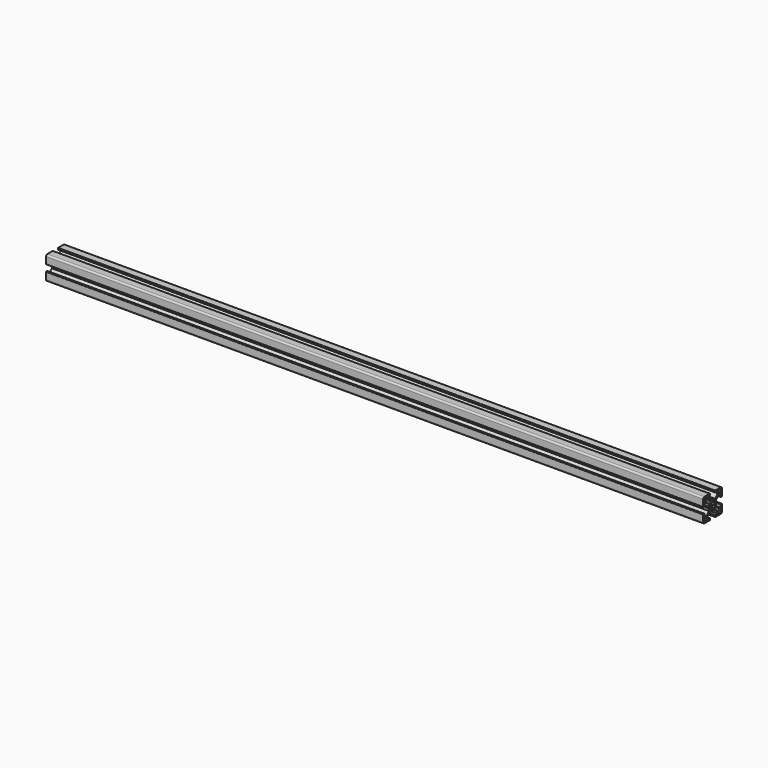
from build123d import *

# Parameters (mm, degrees)
F1_DEPTH = 420


# Not quite as in the source:
# - ends of sketch curves that miss each other by under 0.0002 mm in the source are joined


with BuildPart() as f1:
    # F0 (on Right) → F1 (new body, symmetric)
    with BuildSketch(Plane.YZ):
        with BuildLine():
            Line((14.49994, -4), (13.242475, -4))
            ThreePointArc((13.242475, -4), (12.8889216094, -4.1464466094), (12.742475, -4.5))
            Line((12.742475, -4.5), (12.742475, -7.732519))
            ThreePointArc((12.742475, -7.732519), (12.602449566, -8.0972966877), (12.242781, -8.249967))
            Line((12.242781, -8.249967), (10.260188, -8.249967))
            ThreePointArc((10.260188, -8.249967), (10.0688470492, -8.2119069185), (9.9066360236, -8.1035209764))
            Line((9.9066360236, -8.1035209764), (5.981118, -4.178003))
            ThreePointArc((5.981118, -4.178003), (5.8727320815, -4.0157919508), (5.834672, -3.824451))
            Line((5.834672, -3.824451), (5.834672, -1.012496))
            Line((5.834672, -1.012496), (5.324674, -0.0625))
            Line((5.324674, -0.0625), (5.834672, 0.887496))
            Line((5.834672, 0.887496), (5.834672, 3.824451))
            ThreePointArc((5.834672, 3.824451), (5.8727320815, 4.0157919508), (5.9811180236, 4.1780029764))
            Line((5.9811180236, 4.1780029764), (9.906636, 8.103521))
            ThreePointArc((9.906636, 8.103521), (10.0688470492, 8.2119069185), (10.260188, 8.249967))
            Line((10.260188, 8.249967), (12.242781, 8.249967))
            ThreePointArc((12.242781, 8.249967), (12.602449566, 8.0972966877), (12.7424744042, 7.7325190208))
            Line((12.7424744042, 7.7325190208), (12.742475, 4.5))
            ThreePointArc((12.742475, 4.5), (12.8889216094, 4.1464466094), (13.242475, 4))
            Line((13.242475, 4), (14.49994, 4))
            ThreePointArc((14.49994, 4), (14.8534933906, 4.1464466094), (14.99994, 4.5))
            Line((14.99994, 4.5), (14.99994, 12.999948))
            ThreePointArc((14.99994, 12.999948), (14.4141559055, 14.4141559055), (12.999948, 14.99994))
            Line((12.999948, 14.99994), (4.5, 14.99994))
            ThreePointArc((4.5, 14.99994), (4.1464466094, 14.8534933906), (4, 14.49994))
            Line((4, 14.49994), (4, 13.242475))
            ThreePointArc((4, 13.242475), (4.1464466094, 12.8889216094), (4.5, 12.742475))
            Line((4.5, 12.742475), (7.732519, 12.742475))
            ThreePointArc((7.732519, 12.742475), (8.0972966877, 12.602449566), (8.249967, 12.242781))
            Line((8.249967, 12.242781), (8.249967, 10.260188))
            ThreePointArc((8.249967, 10.260188), (8.2119069185, 10.0688470492), (8.1035209764, 9.9066360236))
            Line((8.1035209764, 9.9066360236), (4.178003, 5.981118))
            ThreePointArc((4.178003, 5.981118), (4.0157919508, 5.8727320815), (3.824451, 5.834672))
            Line((3.824451, 5.834672), (0.949996, 5.834672))
            Line((0.949996, 5.834672), (0, 5.324674))
            Line((0, 5.324674), (-0.949996, 5.834672))
            Line((-0.949996, 5.834672), (-3.824451, 5.834672))
            ThreePointArc((-3.824451, 5.834672), (-4.0157919508, 5.8727320815), (-4.1780029764, 5.9811180236))
            Line((-4.1780029764, 5.9811180236), (-8.103521, 9.906636))
            ThreePointArc((-8.103521, 9.906636), (-8.2119069185, 10.0688470492), (-8.249967, 10.260188))
            Line((-8.249967, 10.260188), (-8.249967, 12.242781))
            ThreePointArc((-8.249967, 12.242781), (-8.0972966877, 12.602449566), (-7.7325190208, 12.7424744042))
            Line((-7.7325190208, 12.7424744042), (-4.5, 12.742475))
            ThreePointArc((-4.5, 12.742475), (-4.1464466094, 12.8889216094), (-4, 13.242475))
            Line((-4, 13.242475), (-4, 14.49994))
            ThreePointArc((-4, 14.49994), (-4.1464466094, 14.8534933906), (-4.5, 14.99994))
            Line((-4.5, 14.99994), (-12.999948, 14.99994))
            ThreePointArc((-12.999948, 14.99994), (-14.4141559055, 14.4141559055), (-14.99994, 12.999948))
            Line((-14.99994, 12.999948), (-14.99994, 4.5))
            ThreePointArc((-14.99994, 4.5), (-14.8534933906, 4.1464466094), (-14.49994, 4))
            Line((-14.49994, 4), (-13.242475, 4))
            ThreePointArc((-13.242475, 4), (-12.8889216094, 4.1464466094), (-12.742475, 4.5))
            Line((-12.742475, 4.5), (-12.742475, 7.732519))
            ThreePointArc((-12.742475, 7.732519), (-12.602449566, 8.0972966877), (-12.242781, 8.249967))
            Line((-12.242781, 8.249967), (-10.260188, 8.249967))
            ThreePointArc((-10.260188, 8.249967), (-10.0688470492, 8.2119069185), (-9.9066360236, 8.1035209764))
            Line((-9.9066360236, 8.1035209764), (-5.981118, 4.178003))
            ThreePointArc((-5.981118, 4.178003), (-5.8727320815, 4.0157919508), (-5.834672, 3.824451))
            Line((-5.834672, 3.824451), (-5.834672, 0.887496))
            Line((-5.834672, 0.887496), (-5.324674, -0.0625))
            Line((-5.324674, -0.0625), (-5.834672, -1.012496))
            Line((-5.834672, -1.012496), (-5.834672, -3.824451))
            ThreePointArc((-5.834672, -3.824451), (-5.8727320815, -4.0157919508), (-5.9811180236, -4.1780029764))
            Line((-5.9811180236, -4.1780029764), (-9.906636, -8.103521))
            ThreePointArc((-9.906636, -8.103521), (-10.0688470492, -8.2119069185), (-10.260188, -8.249967))
            Line((-10.260188, -8.249967), (-12.242781, -8.249967))
            ThreePointArc((-12.242781, -8.249967), (-12.602449566, -8.0972966877), (-12.7424744042, -7.7325190208))
            Line((-12.7424744042, -7.7325190208), (-12.742475, -4.5))
            ThreePointArc((-12.742475, -4.5), (-12.8889216094, -4.1464466094), (-13.242475, -4))
            Line((-13.242475, -4), (-14.49994, -4))
            ThreePointArc((-14.49994, -4), (-14.8534933906, -4.1464466094), (-14.99994, -4.5))
            Line((-14.99994, -4.5), (-14.99994, -12.999948))
            ThreePointArc((-14.99994, -12.999948), (-14.4141559055, -14.4141559055), (-12.999948, -14.99994))
            Line((-12.999948, -14.99994), (-4.5, -14.99994))
            ThreePointArc((-4.5, -14.99994), (-4.1464466094, -14.8534933906), (-4, -14.49994))
            Line((-4, -14.49994), (-4, -13.242475))
            ThreePointArc((-4, -13.242475), (-4.1464466094, -12.8889216094), (-4.5, -12.742475))
            Line((-4.5, -12.742475), (-7.732519, -12.742475))
            ThreePointArc((-7.732519, -12.742475), (-8.0972966877, -12.602449566), (-8.249967, -12.242781))
            Line((-8.249967, -12.242781), (-8.249967, -10.260188))
            ThreePointArc((-8.249967, -10.260188), (-8.2119069185, -10.0688470492), (-8.1035209764, -9.9066360236))
            Line((-8.1035209764, -9.9066360236), (-4.178003, -5.981118))
            ThreePointArc((-4.178003, -5.981118), (-4.0157919508, -5.8727320815), (-3.824451, -5.834672))
            Line((-3.824451, -5.834672), (-0.949996, -5.834672))
            Line((-0.949996, -5.834672), (0, -5.324674))
            Line((0, -5.324674), (0.949996, -5.834672))
            Line((0.949996, -5.834672), (3.824451, -5.834672))
            ThreePointArc((3.824451, -5.834672), (4.0157919508, -5.8727320815), (4.1780029764, -5.9811180236))
            Line((4.1780029764, -5.9811180236), (8.103521, -9.906636))
            ThreePointArc((8.103521, -9.906636), (8.2119069185, -10.0688470492), (8.249967, -10.260188))
            Line((8.249967, -10.260188), (8.249967, -12.242781))
            ThreePointArc((8.249967, -12.242781), (8.0972966877, -12.602449566), (7.7325190208, -12.7424744042))
            Line((7.7325190208, -12.7424744042), (4.5, -12.742475))
            ThreePointArc((4.5, -12.742475), (4.1464466094, -12.8889216094), (4, -13.242475))
            Line((4, -13.242475), (4, -14.49994))
            ThreePointArc((4, -14.49994), (4.1464466094, -14.8534933906), (4.5, -14.99994))
            Line((4.5, -14.99994), (12.999948, -14.99994))
            ThreePointArc((12.999948, -14.99994), (14.4141559055, -14.4141559055), (14.99994, -12.999948))
            Line((14.99994, -12.999948), (14.99994, -4.5))
            ThreePointArc((14.99994, -4.5), (14.8534933906, -4.1464466094), (14.49994, -4))
        make_face()
        with BuildLine():
            ThreePointArc((-13.699945, -9.88096), (-13.5883532694, -9.6115537306), (-13.318947, -9.499962))
            Line((-13.318947, -9.499962), (-9.87996, -9.499962))
            ThreePointArc((-9.87996, -9.499962), (-9.6112608374, -9.6112608374), (-9.499962, -9.87996))
            Line((-9.499962, -9.87996), (-9.499962, -13.318947))
            ThreePointArc((-9.499962, -13.318947), (-9.6115537306, -13.5883532694), (-9.88096, -13.699945))
            Line((-9.88096, -13.699945), (-12.699949, -13.699945))
            ThreePointArc((-12.699949, -13.699945), (-13.4070529528, -13.4070529528), (-13.699945, -12.699949))
            Line((-13.699945, -12.699949), (-13.699945, -9.88096))
        make_face(mode=Mode.SUBTRACT)
        with BuildLine():
            ThreePointArc((9.88096, -13.699945), (9.6115537306, -13.5883532694), (9.499962, -13.318947))
            Line((9.499962, -13.318947), (9.499962, -9.87996))
            ThreePointArc((9.499962, -9.87996), (9.6112608374, -9.6112608374), (9.87996, -9.499962))
            Line((9.87996, -9.499962), (13.318947, -9.499962))
            ThreePointArc((13.318947, -9.499962), (13.5883532694, -9.6115537306), (13.699945, -9.88096))
            Line((13.699945, -9.88096), (13.699945, -12.699949))
            ThreePointArc((13.699945, -12.699949), (13.4070529528, -13.4070529528), (12.699949, -13.699945))
            Line((12.699949, -13.699945), (9.88096, -13.699945))
        make_face(mode=Mode.SUBTRACT)
        with BuildLine():
            ThreePointArc((-9.88096, 13.699945), (-9.6115537306, 13.5883532694), (-9.499962, 13.318947))
            Line((-9.499962, 13.318947), (-9.499962, 9.87996))
            ThreePointArc((-9.499962, 9.87996), (-9.6112608374, 9.6112608374), (-9.87996, 9.499962))
            Line((-9.87996, 9.499962), (-13.318947, 9.499962))
            ThreePointArc((-13.318947, 9.499962), (-13.5883532694, 9.6115537306), (-13.699945, 9.88096))
            Line((-13.699945, 9.88096), (-13.699945, 12.699949))
            ThreePointArc((-13.699945, 12.699949), (-13.4070529528, 13.4070529528), (-12.699949, 13.699945))
            Line((-12.699949, 13.699945), (-9.88096, 13.699945))
        make_face(mode=Mode.SUBTRACT)
        with BuildLine():
            ThreePointArc((1.4942249848, -3.1981389674), (0, -3.529986), (-1.4942249848, -3.1981389674))
            Line((-1.4942249848, -3.1981389674), (-2.473342, -3.979927))
            ThreePointArc((-2.473342, -3.979927), (-3.9002278628, -3.9002278628), (-3.9799273803, -2.4733416963))
            Line((-3.9799273803, -2.4733416963), (-3.198139, -1.494225))
            ThreePointArc((-3.198139, -1.494225), (-3.529986, 0), (-3.1981389674, 1.4942249848))
            Line((-3.1981389674, 1.4942249848), (-3.979927, 2.473342))
            ThreePointArc((-3.979927, 2.473342), (-3.9002278628, 3.9002278628), (-2.4733416963, 3.9799273803))
            Line((-2.4733416963, 3.9799273803), (-1.494225, 3.198139))
            ThreePointArc((-1.494225, 3.198139), (0, 3.529986), (1.4942249848, 3.1981389674))
            Line((1.4942249848, 3.1981389674), (2.473342, 3.979927))
            ThreePointArc((2.473342, 3.979927), (3.9002278628, 3.9002278628), (3.9799273803, 2.4733416963))
            Line((3.9799273803, 2.4733416963), (3.198139, 1.494225))
            ThreePointArc((3.198139, 1.494225), (3.529986, 0), (3.1981389674, -1.4942249848))
            Line((3.1981389674, -1.4942249848), (3.979927, -2.473342))
            ThreePointArc((3.979927, -2.473342), (3.9002278628, -3.9002278628), (2.4733416963, -3.9799273803))
            Line((2.4733416963, -3.9799273803), (1.4942249848, -3.1981389674))
        make_face(mode=Mode.SUBTRACT)
        with BuildLine():
            ThreePointArc((9.499962, 13.318947), (9.6115537306, 13.5883532694), (9.88096, 13.699945))
            Line((9.88096, 13.699945), (12.699949, 13.699945))
            ThreePointArc((12.699949, 13.699945), (13.4070529528, 13.4070529528), (13.699945, 12.699949))
            Line((13.699945, 12.699949), (13.699945, 9.88096))
            ThreePointArc((13.699945, 9.88096), (13.5883532694, 9.6115537306), (13.318947, 9.499962))
            Line((13.318947, 9.499962), (9.87996, 9.499962))
            ThreePointArc((9.87996, 9.499962), (9.6112608374, 9.6112608374), (9.499962, 9.87996))
            Line((9.499962, 9.87996), (9.499962, 13.318947))
        make_face(mode=Mode.SUBTRACT)
    extrude(amount=F1_DEPTH, both=True)


solid = f1.part
